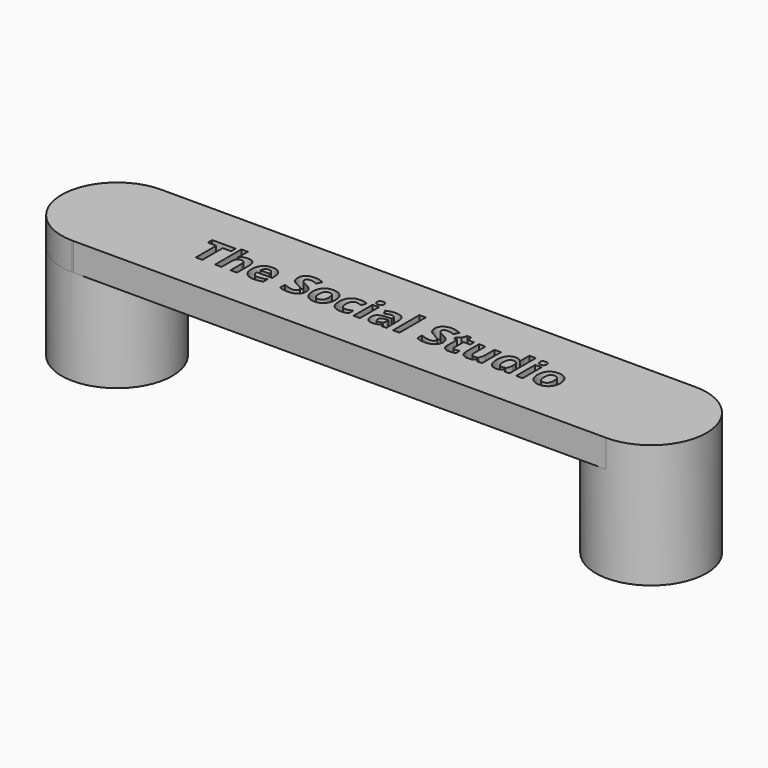
from build123d import *

# Parameters (mm, degrees)
F0_R         = 9.95
F1_DEPTH     = 17.2
F1_FACE_R    = 9.95
F1_FACE1_R   = 9.95
F3_DEPTH     = 5
F4_TEXT_SIZE = 7.7973861035
F5_DEPTH     = 2


# Not quite as in the source:
# - Text() gives the source's letters only with a copy of the font that has no kerning and outlines rounded to 1/6400 em; it was checked with that copy


with BuildPart() as f1:
    # F0 (on Top) → F1 (new body)
    with BuildSketch(Plane.XY):
        with Locations((-48, 0)):
            Circle(F0_R)
    extrude(amount=F1_DEPTH)



with BuildPart() as f1b:
    # F0 (on Top) → F1, piece 2 (new body)
    with BuildSketch(Plane.XY):
        with Locations((48, 0)):
            Circle(F0_R)
    extrude(amount=F1_DEPTH)


with BuildPart() as f1_1:
    add(f1.part)

    add(f1b.part)  # F3 merges F1b
    # F2 (on face) + F1_face (on face) + F1_face1 (on face) → F3 (join)
    with BuildSketch(Plane.XY.offset(17.2)):
        with BuildLine():
            ThreePointArc((-48.1587557759, 9.9487334171), (-57.95, 0), (-48.1587557759, -9.9487334171))
            Line((-48.1587557759, -9.9487334171), (-48.1587557759, 9.9487334171))
        make_face()
        with BuildLine():
            ThreePointArc((-38.05, 0), (-40.9083810039, -6.9793581377), (-47.8412442241, -9.9487334171))
            Line((-47.8412442241, -9.9487334171), (48.1587557759, -9.9487334171))
            Line((48.1587557759, -9.9487334171), (48.1587557759, 9.9487334171))
            Line((48.1587557759, 9.9487334171), (-47.8412442241, 9.9487334171))
            ThreePointArc((-47.8412442241, 9.9487334171), (-40.9083810039, 6.9793581377), (-38.05, 0))
        make_face()
        with BuildLine():
            Line((-48.1587557759, 9.9487334171), (-48.1587557759, -9.9487334171))
            Line((-48.1587557759, -9.9487334171), (-47.8412442241, -9.9487334171))
            ThreePointArc((-47.8412442241, -9.9487334171), (-40.9083810039, -6.9793581377), (-38.05, 0))
            ThreePointArc((-38.05, 0), (-40.9083810039, 6.9793581377), (-47.8412442241, 9.9487334171))
            Line((-47.8412442241, 9.9487334171), (-48.1587557759, 9.9487334171))
        make_face()
        with BuildLine():
            ThreePointArc((-47.8412442241, 9.9487334171), (-48, 9.95), (-48.1587557759, 9.9487334171))
            Line((-48.1587557759, 9.9487334171), (-47.8412442241, 9.9487334171))
        make_face()
        with BuildLine():
            Line((-47.8412442241, -9.9487334171), (-48.1587557759, -9.9487334171))
            ThreePointArc((-48.1587557759, -9.9487334171), (-48, -9.95), (-47.8412442241, -9.9487334171))
        make_face()
    with BuildSketch(Plane(origin=(-48, 0, 17.2), x_dir=(1, 0, 0), z_dir=(0, 0, 1))):
        with Locations((96, 0)):
            Circle(F1_FACE_R)
        Circle(F1_FACE_R)
    with BuildSketch(Plane(origin=(48, 0, 0), x_dir=(1, 0, 0), z_dir=(0, 0, -1))):
        Circle(F1_FACE1_R)
        with Locations((-96, 0)):
            Circle(F1_FACE1_R)
    extrude(amount=F3_DEPTH, dir=(0, 0, 1))

    # F4 (on face) → F5 (cut)
    with BuildSketch(Plane.XY.offset(22.2)):
        with Locations((-33.0012795788, -3.1215900804)):
            Text('The Social Studio', F4_TEXT_SIZE, font='Open Sans', font_style=FontStyle.BOLD, text_align=(TextAlign.LEFT, TextAlign.BOTTOM))
    extrude(amount=-F5_DEPTH, mode=Mode.SUBTRACT)


solid = f1_1.part
